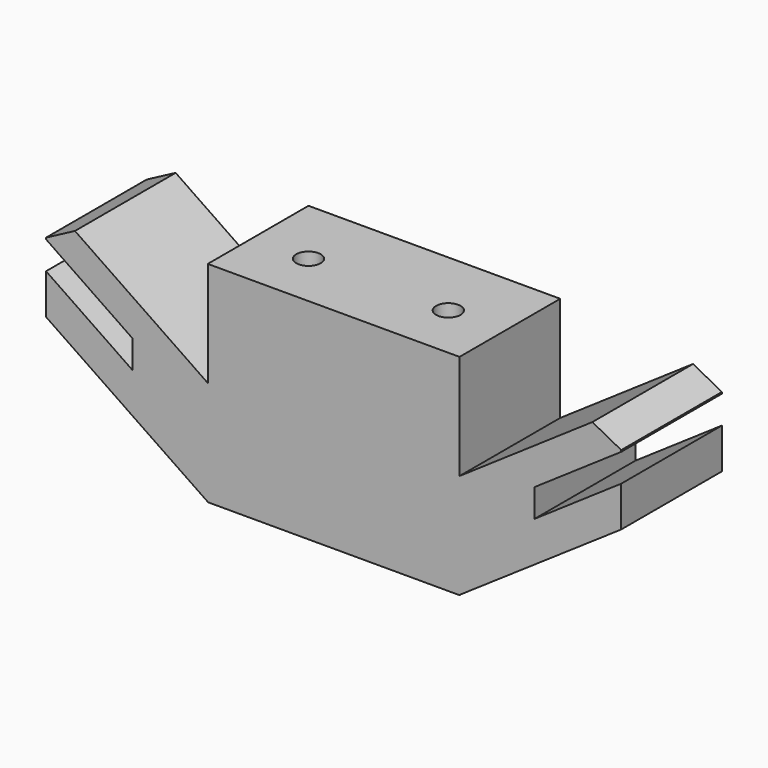
from build123d import *

# Parameters (mm, degrees)
F0_W           = 36
F0_H           = 18
F1_DEPTH       = 15
F3_DEPTH       = 18
F4_DEPTH       = 15
F5_SIZE        = 5
F6_D           = 3.5
F6_CBORE_D     = 10
F6_CBORE_DEPTH = 20


# Not quite as in the source:
# - a feature names something its author has since deleted; it is built from what else it names


with BuildPart() as f1:
    # F0 (on Top) → F1 (new body)
    with BuildSketch(Plane.XY):
        with Locations((0, -9)):
            Rectangle(F0_W, F0_H)
    extrude(amount=F1_DEPTH)

    # F2 (on Front) → F3 (join)
    with BuildSketch(Plane.XZ):
        Polygon((-17.9443880916, 0), (-18, 15), (-41.1238394028, 30.7888584537), (-41.1238394028, 25.5634840578), (-28.7360682942, 17.105167029), (-28.7360682942, 13.1013058126), (-41.1238394028, 21.5596228414), (-41.1238394028, 15.7888584537), align=None)
        Polygon((28.7360682942, 17.105167029), (41.1238394028, 25.5634840578), (41.1238394028, 30.7888584537), (18, 15), (17.9443880916, 0), (41.1238394028, 15.7888584537), (41.1238394028, 21.5596228414), (28.7360682942, 13.1013058126), align=None)
    extrude(amount=F3_DEPTH)

    # F4 (add): a face of the model
    f4_faces = [f1.faces().sort_by_distance(p)[0] for p in [
        (0, -9, 15),
    ]]
    extrude(f4_faces, amount=F4_DEPTH)

    # F5
    f5_edges = [f1.edges().sort_by_distance(p)[0] for p in [
        (41.123839, -9, 30.788858),
        (-41.123839, -9, 30.788858),
    ]]
    chamfer(f5_edges, length=F5_SIZE)

    # F6 (through all)
    with Locations(Plane(origin=(0, 0, 0), x_dir=(1, 0, 0), z_dir=(0, 0, -1))):
        with Locations((-10, 10), (10, 10)):
            CounterBoreHole(F6_D / 2, F6_CBORE_D / 2, F6_CBORE_DEPTH)


solid = f1.part
